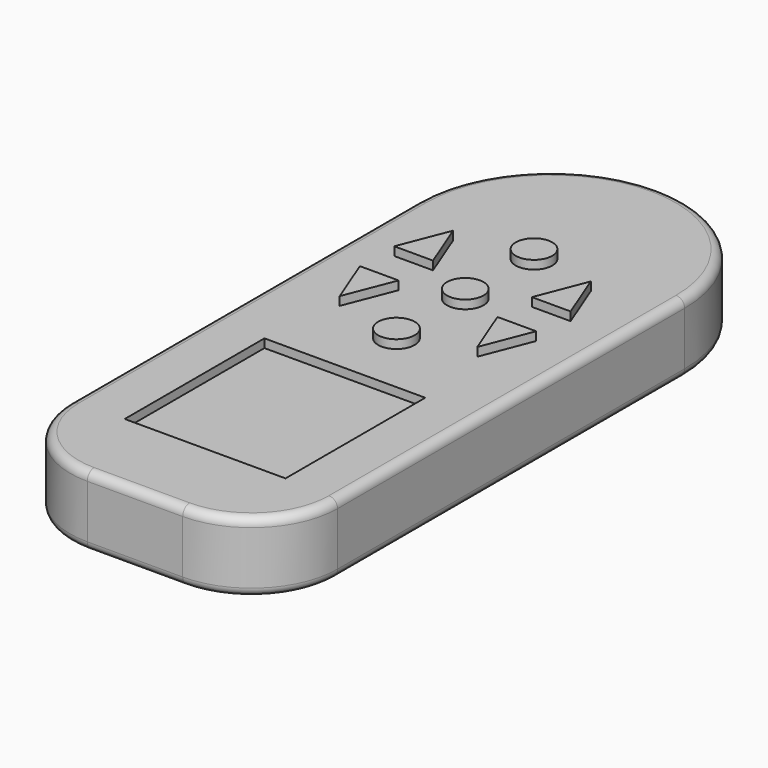
from build123d import *

# Parameters (mm, degrees)
F0_W     = 62.2
F0_H     = 152
F1_DEPTH = 16.38
F2_R     = 20
F3_R     = 31.09999
F4_R     = 2
F5_W     = 37.4
F5_H     = 40.62
F6_DEPTH = 2
F7_R     = 4.25
F8_DEPTH = 2


# Not quite as in the source:
# - a fillet or chamfer is up to 0.001 mm smaller than in the source, because OpenCascade refuses the exact size


with BuildPart() as f1:
    # F0 (on Top) → F1 (new body)
    with BuildSketch(Plane.XY):
        Rectangle(F0_W, F0_H)
    extrude(amount=F1_DEPTH)

    # F2
    f2_edges = [f1.edges().sort_by_distance(p)[0] for p in [
        (-31.1, -76, 8.19),
        (31.1, -76, 8.19),
    ]]
    fillet(f2_edges, radius=F2_R)

    # F3 (radius 31.1 in the source; OpenCascade refuses exactly that, so slightly less here)
    f3_edges = [f1.edges().sort_by_distance(p)[0] for p in [
        (31.1, 76, 8.19),
        (-31.1, 76, 8.19),
    ]]
    fillet(f3_edges, radius=F3_R)

    # F4
    f4_edges = [f1.edges().sort_by_distance(p)[0] for p in [
        (31.1, -5.549995, 16.38),
        (31.1, -5.549995, 0),
    ]]
    fillet(f4_edges, radius=F4_R)

    # F5 (on face) → F6 (cut)
    with BuildSketch(Plane.XY.offset(16.38)):
        with Locations((0, -35.31)):
            Rectangle(F5_W, F5_H)
    extrude(amount=-F6_DEPTH, mode=Mode.SUBTRACT)

    # F7 (on face) → F8 (join)
    with BuildSketch(Plane.XY.offset(16.38)):
        Polygon((11.5, 15), (16, 3.5), (20.5, 15), align=None)
        Circle(F7_R)
        Polygon((-16, 3.5), (-11.5, 15), (-20.5, 15), align=None)
        Polygon((-20.5, 25), (-11.5, 25), (-16, 36.5), align=None)
        with Locations((0, 20)):
            Circle(F7_R)
        Polygon((11.5, 25), (20.5, 25), (16, 36.5), align=None)
        with Locations((0, 40)):
            Circle(F7_R)
    extrude(amount=F8_DEPTH)


solid = f1.part
